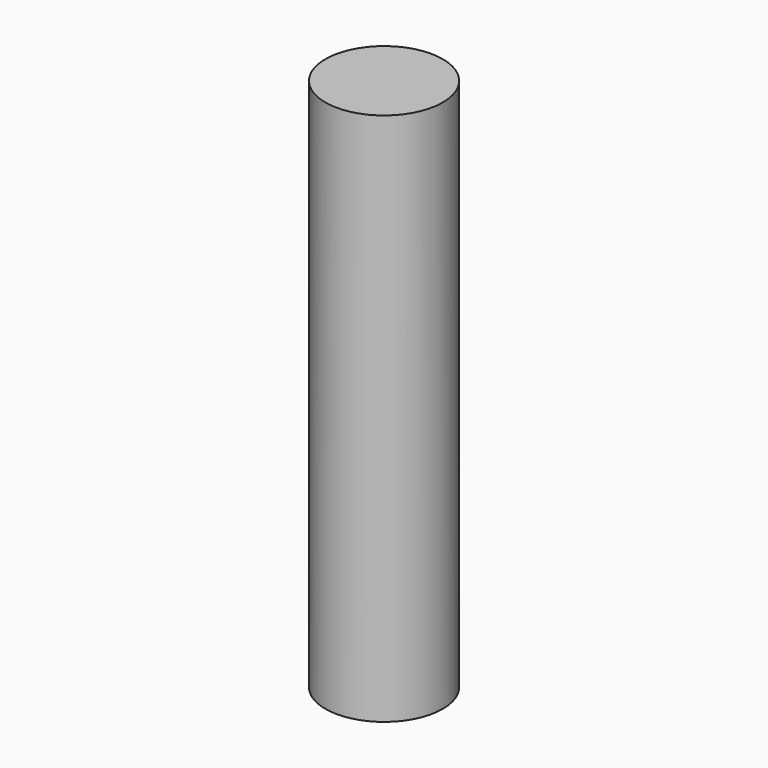
from build123d import *

# Parameters (mm, degrees)
F0_R     = 15.5013046097
F1_DEPTH = 140.97


# Not quite as in the source:
# - the program builds the solid bodies; features that only make, move or delete a surface that nothing else refers to are left out


with BuildPart() as f1:
    # F0 (on Top) → F1 (new body)
    with BuildSketch(Plane.XY):
        with Locations((0, 44.4700233638)):
            Circle(F0_R)
    extrude(amount=-F1_DEPTH)


solid = f1.part
